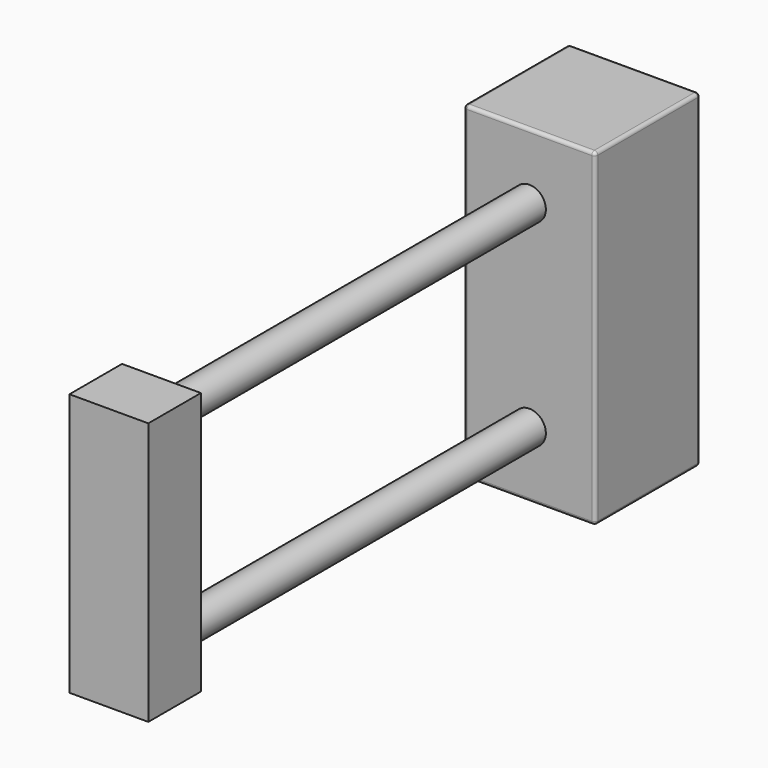
from build123d import *

# Parameters (mm, degrees)
F0_W     = 20
F0_H     = 50
F1_DEPTH = 20
F2_R     = 0.508
F3_R     = 2.5
F4_DEPTH = 70
F5_W     = 12
F5_H     = 40
F5_R     = 2.5
F6_DEPTH = 10


# Not quite as in the source:
# - a feature names something its author has since deleted; it is built from what else it names


with BuildPart() as f1:
    # F0 (on Front) → F1 (new body)
    with BuildSketch(Plane.XZ):
        with Locations((0, 15)):
            Rectangle(F0_W, F0_H)
    extrude(amount=F1_DEPTH)

    # F2
    f2_edges = [f1.edges().sort_by_distance(p)[0] for p in [
        (0, -20, 40),
        (-10, -20, 15),
        (0, -20, -10),
        (10, -20, 15),
        (10, -10, -10),
        (10, -10, 40),
        (10, 0, 15),
        (-10, -10, 40),
        (0, 0, 40),
        (-10, -10, -10),
        (-10, 0, 15),
        (0, 0, -10),
    ]]
    fillet(f2_edges, radius=F2_R)

    # F3 (on face) → F4 (join)
    with BuildSketch(Plane.XZ.offset(20)):
        with Locations((0, 30)):
            Circle(F3_R)
        Circle(F3_R)
    extrude(amount=F4_DEPTH)

    # F5 (on face) → F6 (join)
    with BuildSketch(Plane.XZ.offset(90)):
        with Locations((0, 15)):
            Rectangle(F5_W, F5_H)
        with Locations((0, 30)):
            Circle(F5_R, mode=Mode.SUBTRACT)
        with Locations((0, 30)):
            Circle(F5_R)
    extrude(amount=F6_DEPTH)


solid = f1.part
